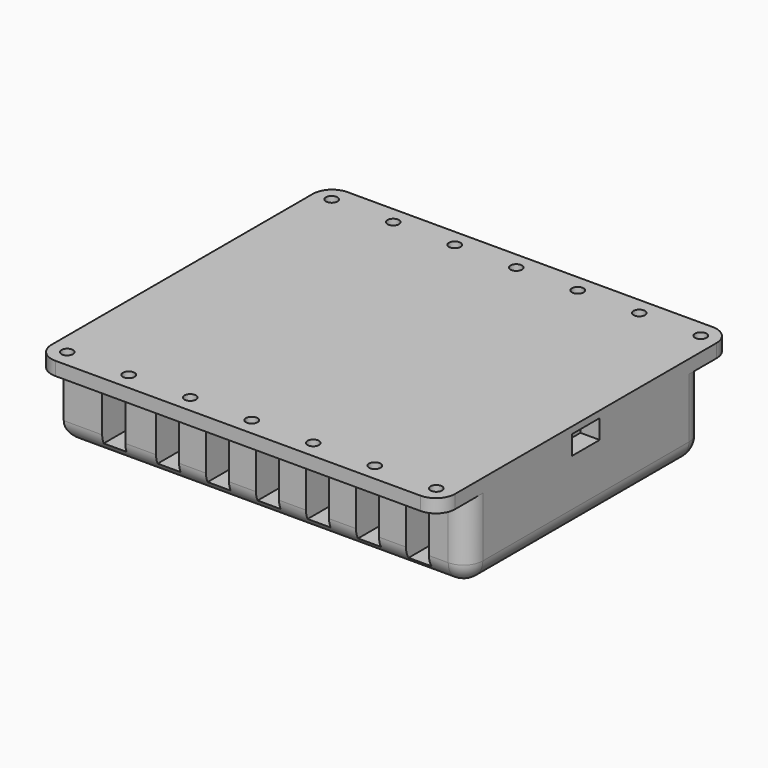
from build123d import *

# Parameters (mm, degrees)
F0_W          = 105
F0_H          = 95
F1_DEPTH      = 1.75
F2_W          = 105
F2_H          = 77
F3_DEPTH      = 20.5
F4_W          = 54
F4_H          = 21
F5_DEPTH      = 9
F6_W          = 9
F6_H          = 5
F7_DEPTH      = 5
F8_W          = 21
F8_H          = 13
F9_DEPTH      = 1
F11_D         = 3
F13_D         = 3
F14_W         = 6
F14_H         = 15
F15_DEPTH     = 25
F16_T1_DEPTH  = 67
F16_T3_DEPTH  = 100
F16_T5_DEPTH  = 15.5
F16_T7_DEPTH  = 49
F16_T9_DEPTH  = 11
F16_T11_DEPTH = 21
F16_T13_DEPTH = 4
F16_T15_DEPTH = 77
F16_S19_W     = 5.1
F16_S19_H     = 5.1
F16_T20_DEPTH = 5.1
F16_S25_W     = 5.1
F16_S25_H     = 5.1
F16_T26_DEPTH = 5.1
F16_S31_W     = 5.1
F16_S31_H     = 5.1
F16_T32_DEPTH = 5.1
F16_S37_W     = 5.1
F16_S37_H     = 5.1
F16_T38_DEPTH = 5.1
F16_T45_DEPTH = 89.5
F16_T49_DEPTH = 112.5
F16_T56_DEPTH = 61.5
F16_T60_DEPTH = 33.5
F16_T67_DEPTH = 33.5
F16_T71_DEPTH = 61.5
F16_T78_DEPTH = 89.5
F16_T82_DEPTH = 112.5
F17_R         = 5


# Not quite as in the source:
# - a fillet or chamfer that OpenCascade refuses, or shapes differently, is made with other operations: its cross-section is extruded or revolved along the edge and cut away or added
# - two fillets or chamfers of one size are made in one step


with BuildPart() as f1:
    # F0 (on Top) → F1 (new body, symmetric)
    with BuildSketch(Plane.XY):
        with Locations((-0.3900006413, 10.040976562)):
            Rectangle(F0_W, F0_H)
    extrude(amount=F1_DEPTH, both=True)

    # F2 (on face) → F3 (join)
    with BuildSketch(Plane(origin=(0, 0, -1.75), x_dir=(1, 0, 0), z_dir=(0, 0, -1))):
        with Locations((-0.3900006413, -10.040976562)):
            Rectangle(F2_W, F2_H)
    extrude(amount=F3_DEPTH)

    # F4 (on face) → F5 (join)
    with BuildSketch(Plane(origin=(0, 0, -22.25), x_dir=(1, 0, 0), z_dir=(0, 0, -1))):
        with Locations((14.1099993587, -33.040976562)):
            Rectangle(F4_W, F4_H)
    extrude(amount=F5_DEPTH)

    # F6 (on face) → F7 (cut)
    with BuildSketch(Plane.YZ.offset(52.1099993587)):
        with Locations((10.040976562, -2.5)):
            Rectangle(F6_W, F6_H)
    extrude(amount=-F7_DEPTH, mode=Mode.SUBTRACT)

    # F8 (on face) → F9 (join)
    with BuildSketch(Plane(origin=(-52.8900006413, 0, 0), x_dir=(0, -1, 0), z_dir=(-1, 0, 0))):
        with Locations((-10.040976562, -6.5)):
            Rectangle(F8_W, F8_H)
    extrude(amount=F9_DEPTH)

    # F11 (through all)
    with Locations(Plane(origin=(0, 0, -1.75), x_dir=(1, 0, 0), z_dir=(0, 0, -1))):
        with Locations((47.6099993587, 32.959023438), (31.6099993587, 32.959023438), (15.6099993587, 32.959023438), (-0.3900006413, 32.959023438), (-16.3900006413, 32.959023438), (-32.3900006413, 32.959023438), (-48.3900006413, 32.959023438)):
            Hole(F11_D / 2)

    # F13 (through all)
    with Locations(Plane(origin=(0, 0, -1.75), x_dir=(1, 0, 0), z_dir=(0, 0, -1))):
        with Locations((47.6099993587, -53.040976562), (31.6099993587, -53.040976562), (15.6099993587, -53.040976562), (-0.3900006413, -53.040976562), (-16.3900006413, -53.040976562), (-32.3900006413, -53.040976562), (-48.3900006413, -53.040976562)):
            Hole(F13_D / 2)

    # F14 (on face) → F15 (cut)
    with BuildSketch(Plane.XZ.offset(28.459023438)):
        with Locations((-39.8900006413, -11.9078365183)):
            Rectangle(F14_W, F14_H)
        with Locations((-25.8900006413, -12.0000001043)):
            Rectangle(F14_W, F14_H)
        with Locations((-12.8900006413, -11.9999996386)):
            Rectangle(F14_W, F14_H)
        with Locations((0.1099993587, -11.999999173)):
            Rectangle(F14_W, F14_H)
        with Locations((13.1099993587, -11.9999996386)):
            Rectangle(F14_W, F14_H)
        with Locations((26.1099993587, -12.2822578996)):
            Rectangle(F14_W, F14_H)
        with Locations((39.1099993587, -12.5645168446)):
            Rectangle(F14_W, F14_H)
    extrude(amount=-F15_DEPTH, mode=Mode.SUBTRACT)

    # F16: fillet of radius 5 on 12 edges, made by hand

    # F16_s2 → F16_t1 (cut)
    with BuildSketch(Plane.XZ.offset(-43.540976562)):
        with BuildLine():
            ThreePointArc((52.1099993587, -17.25), (50.6455332646, -20.7855339059), (47.1099993587, -22.25))
            Line((47.1099993587, -22.25), (47.1099993587, -22.35))
            Line((47.1099993587, -22.35), (52.2099993587, -22.35))
            Line((52.2099993587, -22.35), (52.2099993587, -17.25))
            Line((52.2099993587, -17.25), (52.1099993587, -17.25))
        make_face()
    extrude(amount=F16_T1_DEPTH, mode=Mode.SUBTRACT)

    # F16_s4 → F16_t3 (cut)
    with BuildSketch(Plane.YZ.offset(-52.8900006413)):
        with BuildLine():
            ThreePointArc((-23.459023438, -22.25), (-26.9945573439, -20.7855339059), (-28.459023438, -17.25))
            Line((-28.459023438, -17.25), (-28.559023438, -17.25))
            Line((-28.559023438, -17.25), (-28.559023438, -22.35))
            Line((-28.559023438, -22.35), (-23.459023438, -22.35))
            Line((-23.459023438, -22.35), (-23.459023438, -22.25))
        make_face()
        with BuildLine():
            ThreePointArc((48.540976562, -17.25), (47.076510468, -20.7855339059), (43.540976562, -22.25))
            Line((43.540976562, -22.25), (43.540976562, -22.35))
            Line((43.540976562, -22.35), (48.640976562, -22.35))
            Line((48.640976562, -22.35), (48.640976562, -17.25))
            Line((48.640976562, -17.25), (48.540976562, -17.25))
        make_face()
    extrude(amount=F16_T3_DEPTH, mode=Mode.SUBTRACT)

    # F16_s6 → F16_t5 (cut)
    with BuildSketch(Plane.XY.offset(-17.25)):
        with BuildLine():
            ThreePointArc((52.1099993587, -23.459023438), (50.6455332646, -26.9945573439), (47.1099993587, -28.459023438))
            Line((47.1099993587, -28.459023438), (47.1099993587, -28.559023438))
            Line((47.1099993587, -28.559023438), (52.2099993587, -28.559023438))
            Line((52.2099993587, -28.559023438), (52.2099993587, -23.459023438))
            Line((52.2099993587, -23.459023438), (52.1099993587, -23.459023438))
        make_face()
        with BuildLine():
            ThreePointArc((52.1099993587, 43.540976562), (50.6455332646, 47.076510468), (47.1099993587, 48.540976562))
            Line((47.1099993587, 48.540976562), (47.1099993587, 48.640976562))
            Line((47.1099993587, 48.640976562), (52.2099993587, 48.640976562))
            Line((52.2099993587, 48.640976562), (52.2099993587, 43.540976562))
            Line((52.2099993587, 43.540976562), (52.1099993587, 43.540976562))
        make_face()
    extrude(amount=F16_T5_DEPTH, mode=Mode.SUBTRACT)

    # F16_s8 → F16_t7 (cut)
    with BuildSketch(Plane.YZ.offset(-12.8900006413)):
        with BuildLine():
            ThreePointArc((22.540976562, -26.25), (24.0054426561, -29.7855339059), (27.540976562, -31.25))
            Line((27.540976562, -31.25), (27.540976562, -31.35))
            Line((27.540976562, -31.35), (22.440976562, -31.35))
            Line((22.440976562, -31.35), (22.440976562, -26.25))
            Line((22.440976562, -26.25), (22.540976562, -26.25))
        make_face()
        with BuildLine():
            ThreePointArc((43.540976562, -26.25), (42.076510468, -29.7855339059), (38.540976562, -31.25))
            Line((38.540976562, -31.25), (38.540976562, -31.35))
            Line((38.540976562, -31.35), (43.640976562, -31.35))
            Line((43.640976562, -31.35), (43.640976562, -26.25))
            Line((43.640976562, -26.25), (43.540976562, -26.25))
        make_face()
    extrude(amount=F16_T7_DEPTH, mode=Mode.SUBTRACT)

    # F16_s10 → F16_t9 (cut)
    with BuildSketch(Plane.XZ.offset(-38.540976562)):
        with BuildLine():
            ThreePointArc((41.1099993587, -26.25), (39.6455332646, -29.7855339059), (36.1099993587, -31.25))
            Line((36.1099993587, -31.25), (36.1099993587, -31.35))
            Line((36.1099993587, -31.35), (41.2099993587, -31.35))
            Line((41.2099993587, -31.35), (41.2099993587, -26.25))
            Line((41.2099993587, -26.25), (41.1099993587, -26.25))
        make_face()
    extrude(amount=F16_T9_DEPTH, mode=Mode.SUBTRACT)

    # F16_s12 → F16_t11 (cut)
    with BuildSketch(Plane.XZ.offset(-43.540976562)):
        with BuildLine():
            ThreePointArc((-12.8900006413, -26.25), (-11.4255345473, -29.7855339059), (-7.8900006413, -31.25))
            Line((-7.8900006413, -31.25), (-7.8900006413, -31.35))
            Line((-7.8900006413, -31.35), (-12.9900006413, -31.35))
            Line((-12.9900006413, -31.35), (-12.9900006413, -26.25))
            Line((-12.9900006413, -26.25), (-12.8900006413, -26.25))
        make_face()
    extrude(amount=F16_T11_DEPTH, mode=Mode.SUBTRACT)

    # F16_s14 → F16_t13 (cut)
    with BuildSketch(Plane.XY.offset(-26.25)):
        with BuildLine():
            ThreePointArc((36.1099993587, 22.540976562), (39.6455332646, 24.0054426561), (41.1099993587, 27.540976562))
            Line((41.1099993587, 27.540976562), (41.2099993587, 27.540976562))
            Line((41.2099993587, 27.540976562), (41.2099993587, 22.440976562))
            Line((41.2099993587, 22.440976562), (36.1099993587, 22.440976562))
            Line((36.1099993587, 22.440976562), (36.1099993587, 22.540976562))
        make_face()
        with BuildLine():
            ThreePointArc((36.1099993587, 43.540976562), (39.6455332646, 42.076510468), (41.1099993587, 38.540976562))
            Line((41.1099993587, 38.540976562), (41.2099993587, 38.540976562))
            Line((41.2099993587, 38.540976562), (41.2099993587, 43.640976562))
            Line((41.2099993587, 43.640976562), (36.1099993587, 43.640976562))
            Line((36.1099993587, 43.640976562), (36.1099993587, 43.540976562))
        make_face()
    extrude(amount=F16_T13_DEPTH, mode=Mode.SUBTRACT)

    # F16_s16 → F16_t15 (cut)
    with BuildSketch(Plane.XZ.offset(-48.540976562)):
        with BuildLine():
            ThreePointArc((-52.8900006413, -17.25), (-51.4255345473, -20.7855339059), (-47.8900006413, -22.25))
            Line((-47.8900006413, -22.25), (-47.8900006413, -22.35))
            Line((-47.8900006413, -22.35), (-52.9900006413, -22.35))
            Line((-52.9900006413, -22.35), (-52.9900006413, -17.25))
            Line((-52.9900006413, -17.25), (-52.8900006413, -17.25))
        make_face()
    extrude(amount=F16_T15_DEPTH, mode=Mode.SUBTRACT)


with BuildPart() as f16_tool18:
    # F16_s19 → F16_t20 (new body)
    with BuildSketch(Plane.YZ.offset(47.1099993587)):
        with Locations((46.090976562, -19.8)):
            Rectangle(F16_S19_W, F16_S19_H)
    extrude(amount=F16_T20_DEPTH)

    # F16_s21 → F16_t22 (revolve, cut)
    with BuildSketch(Plane(origin=(47.1099993587, 43.540976562, -17.25), x_dir=(0, -0.7071067812, 0.7071067812), z_dir=(0, 0.7071067812, 0.7071067812))):
        with BuildLine():
            ThreePointArc((0, -5), (5, 0), (0, 5))
            Line((0, 5), (0, -5))
        make_face()
    revolve(axis=Axis((47.1099993587, 43.540976562, -17.25), (1, 0, 0)), mode=Mode.SUBTRACT)


with BuildPart() as f1_1:
    add(f1.part)

    # F16_t17: cut F16_tool18
    add(f16_tool18.part, mode=Mode.SUBTRACT)


with BuildPart() as f16_tool24:
    # F16_s25 → F16_t26 (new body)
    with BuildSketch(Plane.XZ.offset(23.459023438)):
        with Locations((49.6599993587, -19.8)):
            Rectangle(F16_S25_W, F16_S25_H)
    extrude(amount=F16_T26_DEPTH)

    # F16_s27 → F16_t28 (revolve, cut)
    with BuildSketch(Plane(origin=(47.1099993587, -23.459023438, -17.25), x_dir=(-0.7071067812, 0, 0.7071067812), z_dir=(0.7071067812, 0, 0.7071067812))):
        with BuildLine():
            ThreePointArc((0, -5), (5, 0), (0, 5))
            Line((0, 5), (0, -5))
        make_face()
    revolve(axis=Axis((47.1099993587, -23.459023438, -17.25), (0, -1, 0)), mode=Mode.SUBTRACT)


with BuildPart() as f1_2:
    add(f1_1.part)

    # F16_t23: cut F16_tool24
    add(f16_tool24.part, mode=Mode.SUBTRACT)


with BuildPart() as f16_tool30:
    # F16_s31 → F16_t32 (new body)
    with BuildSketch(Plane.XZ.offset(-27.540976562)):
        with Locations((38.6599993587, -28.8)):
            Rectangle(F16_S31_W, F16_S31_H)
    extrude(amount=F16_T32_DEPTH)

    # F16_s33 → F16_t34 (revolve, cut)
    with BuildSketch(Plane(origin=(36.1099993587, 27.540976562, -26.25), x_dir=(-0.7071067812, 0, 0.7071067812), z_dir=(0.7071067812, 0, 0.7071067812))):
        with BuildLine():
            ThreePointArc((0, -5), (5, 0), (0, 5))
            Line((0, 5), (0, -5))
        make_face()
    revolve(axis=Axis((36.1099993587, 27.540976562, -26.25), (0, -1, 0)), mode=Mode.SUBTRACT)


with BuildPart() as f1_3:
    add(f1_2.part)

    # F16_t29: cut F16_tool30
    add(f16_tool30.part, mode=Mode.SUBTRACT)


with BuildPart() as f16_tool36:
    # F16_s37 → F16_t38 (new body)
    with BuildSketch(Plane.XY.offset(-26.25)):
        with Locations((38.6599993587, 41.090976562)):
            Rectangle(F16_S37_W, F16_S37_H)
    extrude(amount=-F16_T38_DEPTH)

    # F16_s39 → F16_t40 (revolve, cut)
    with BuildSketch(Plane(origin=(36.1099993587, 38.540976562, -26.25), x_dir=(-0.7071067812, -0.7071067812, 0), z_dir=(0.7071067812, -0.7071067812, 0))):
        with BuildLine():
            ThreePointArc((0, -5), (5, 0), (0, 5))
            Line((0, 5), (0, -5))
        make_face()
    revolve(axis=Axis((36.1099993587, 38.540976562, -26.25), (0, 0, -1)), mode=Mode.SUBTRACT)


with BuildPart() as f1_4:
    add(f1_3.part)

    # F16_t35: cut F16_tool36
    add(f16_tool36.part, mode=Mode.SUBTRACT)


with BuildPart() as f16_tool43:
    # F16_s44 → F16_t45 (new body)
    with BuildSketch(Plane.XZ.offset(40.959023438)):
        with BuildLine():
            ThreePointArc((-52.8900006413, -17.25), (-51.4255345473, -20.7855339059), (-47.8900006413, -22.25))
            Line((-47.8900006413, -22.25), (-47.8900006413, -22.35))
            Line((-47.8900006413, -22.35), (-52.9900006413, -22.35))
            Line((-52.9900006413, -22.35), (-52.9900006413, -17.25))
            Line((-52.9900006413, -17.25), (-52.8900006413, -17.25))
        make_face()
    extrude(amount=-F16_T45_DEPTH)

    split(bisect_by=Plane.XZ.offset(28.459023438), keep=Keep.TOP)


with BuildPart() as f16_tool47:
    # F16_s48 → F16_t49 (new body)
    with BuildSketch(Plane.YZ.offset(47.1099993587)):
        with BuildLine():
            ThreePointArc((-23.459023438, -22.25), (-26.9945573439, -20.7855339059), (-28.459023438, -17.25))
            Line((-28.459023438, -17.25), (-28.559023438, -17.25))
            Line((-28.559023438, -17.25), (-28.559023438, -22.35))
            Line((-28.559023438, -22.35), (-23.459023438, -22.35))
            Line((-23.459023438, -22.35), (-23.459023438, -22.25))
        make_face()
    extrude(amount=-F16_T49_DEPTH)

    split(bisect_by=Plane.YZ.offset(-52.8900006413), keep=Keep.BOTTOM)


with BuildPart() as f16_tool43_1:
    add(f16_tool43.part)

    # F16_t51: intersect F16_tool47
    add(f16_tool47.part, mode=Mode.INTERSECT)


with BuildPart() as f1_5:
    add(f1_4.part)

    # F16_t41: cut F16_tool43
    add(f16_tool43_1.part, mode=Mode.SUBTRACT)


with BuildPart() as f16_tool54:
    # F16_s55 → F16_t56 (new body)
    with BuildSketch(Plane.YZ.offset(36.1099993587)):
        with BuildLine():
            ThreePointArc((22.540976562, -26.25), (24.0054426561, -29.7855339059), (27.540976562, -31.25))
            Line((27.540976562, -31.25), (27.540976562, -31.35))
            Line((27.540976562, -31.35), (22.440976562, -31.35))
            Line((22.440976562, -31.35), (22.440976562, -26.25))
            Line((22.440976562, -26.25), (22.540976562, -26.25))
        make_face()
    extrude(amount=-F16_T56_DEPTH)

    split(bisect_by=Plane.YZ.offset(-12.8900006413), keep=Keep.BOTTOM)


with BuildPart() as f16_tool58:
    # F16_s59 → F16_t60 (new body)
    with BuildSketch(Plane.XZ.offset(-10.040976562)):
        with BuildLine():
            ThreePointArc((-12.8900006413, -26.25), (-11.4255345473, -29.7855339059), (-7.8900006413, -31.25))
            Line((-7.8900006413, -31.25), (-7.8900006413, -31.35))
            Line((-7.8900006413, -31.35), (-12.9900006413, -31.35))
            Line((-12.9900006413, -31.35), (-12.9900006413, -26.25))
            Line((-12.9900006413, -26.25), (-12.8900006413, -26.25))
        make_face()
    extrude(amount=-F16_T60_DEPTH)

    split(bisect_by=Plane.XZ.offset(-22.540976562), keep=Keep.TOP)


with BuildPart() as f16_tool54_1:
    add(f16_tool54.part)

    # F16_t62: intersect F16_tool58
    add(f16_tool58.part, mode=Mode.INTERSECT)


with BuildPart() as f1_6:
    add(f1_5.part)

    # F16_t52: cut F16_tool54
    add(f16_tool54_1.part, mode=Mode.SUBTRACT)


with BuildPart() as f16_tool65:
    # F16_s66 → F16_t67 (new body)
    with BuildSketch(Plane.XZ.offset(-22.540976562)):
        with BuildLine():
            ThreePointArc((-12.8900006413, -26.25), (-11.4255345473, -29.7855339059), (-7.8900006413, -31.25))
            Line((-7.8900006413, -31.25), (-7.8900006413, -31.35))
            Line((-7.8900006413, -31.35), (-12.9900006413, -31.35))
            Line((-12.9900006413, -31.35), (-12.9900006413, -26.25))
            Line((-12.9900006413, -26.25), (-12.8900006413, -26.25))
        make_face()
    extrude(amount=-F16_T67_DEPTH)

    split(bisect_by=Plane.XZ.offset(-43.540976562), keep=Keep.BOTTOM)


with BuildPart() as f16_tool69:
    # F16_s70 → F16_t71 (new body)
    with BuildSketch(Plane.YZ.offset(-25.3900006413)):
        with BuildLine():
            ThreePointArc((43.540976562, -26.25), (42.076510468, -29.7855339059), (38.540976562, -31.25))
            Line((38.540976562, -31.25), (38.540976562, -31.35))
            Line((38.540976562, -31.35), (43.640976562, -31.35))
            Line((43.640976562, -31.35), (43.640976562, -26.25))
            Line((43.640976562, -26.25), (43.540976562, -26.25))
        make_face()
    extrude(amount=F16_T71_DEPTH)

    split(bisect_by=Plane.YZ.offset(-12.8900006413), keep=Keep.BOTTOM)


with BuildPart() as f16_tool65_1:
    add(f16_tool65.part)

    # F16_t73: intersect F16_tool69
    add(f16_tool69.part, mode=Mode.INTERSECT)


with BuildPart() as f1_7:
    add(f1_6.part)

    # F16_t63: cut F16_tool65
    add(f16_tool65_1.part, mode=Mode.SUBTRACT)


with BuildPart() as f16_tool76:
    # F16_s77 → F16_t78 (new body)
    with BuildSketch(Plane.XZ.offset(28.459023438)):
        with BuildLine():
            ThreePointArc((-52.8900006413, -17.25), (-51.4255345473, -20.7855339059), (-47.8900006413, -22.25))
            Line((-47.8900006413, -22.25), (-47.8900006413, -22.35))
            Line((-47.8900006413, -22.35), (-52.9900006413, -22.35))
            Line((-52.9900006413, -22.35), (-52.9900006413, -17.25))
            Line((-52.9900006413, -17.25), (-52.8900006413, -17.25))
        make_face()
    extrude(amount=-F16_T78_DEPTH)

    split(bisect_by=Plane.XZ.offset(-48.540976562), keep=Keep.BOTTOM)


with BuildPart() as f16_tool80:
    # F16_s81 → F16_t82 (new body)
    with BuildSketch(Plane.YZ.offset(-65.3900006413)):
        with BuildLine():
            ThreePointArc((48.540976562, -17.25), (47.076510468, -20.7855339059), (43.540976562, -22.25))
            Line((43.540976562, -22.25), (43.540976562, -22.35))
            Line((43.540976562, -22.35), (48.640976562, -22.35))
            Line((48.640976562, -22.35), (48.640976562, -17.25))
            Line((48.640976562, -17.25), (48.540976562, -17.25))
        make_face()
    extrude(amount=F16_T82_DEPTH)

    split(bisect_by=Plane.YZ.offset(-52.8900006413), keep=Keep.BOTTOM)


with BuildPart() as f16_tool76_1:
    add(f16_tool76.part)

    # F16_t84: intersect F16_tool80
    add(f16_tool80.part, mode=Mode.INTERSECT)


with BuildPart() as f1_8:
    add(f1_7.part)

    # F16_t74: cut F16_tool76
    add(f16_tool76_1.part, mode=Mode.SUBTRACT)

    # F17
    f17_edges = [f1_8.edges().sort_by_distance(p)[0] for p in [
        (-52.890001, 57.540977, 0),
        (52.109999, 57.540977, 0),
        (-52.890001, -37.459023, 0),
        (52.109999, -37.459023, 0),
    ]]
    fillet(f17_edges, radius=F17_R)


solid = f1_8.part
